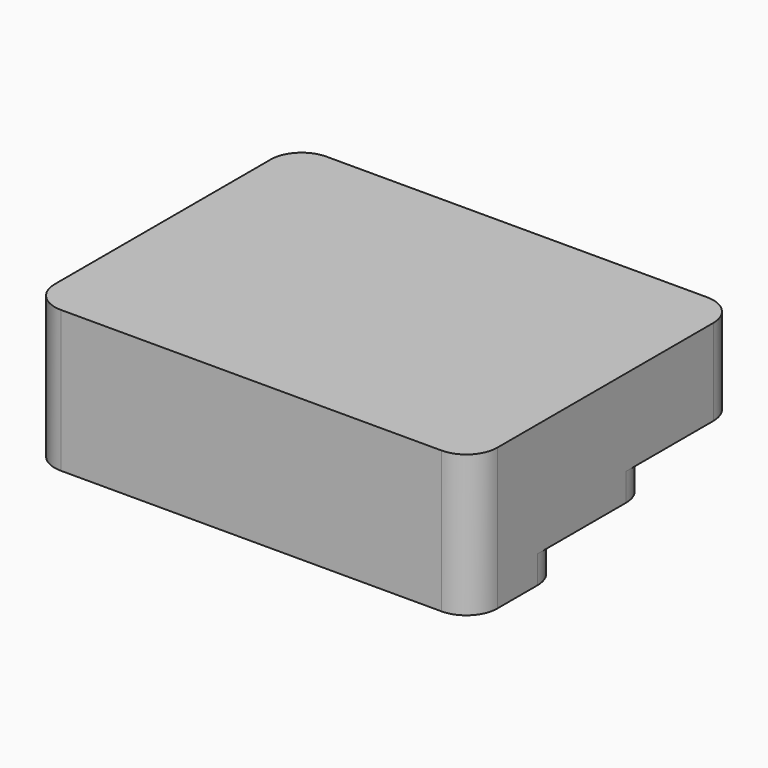
from build123d import *

# Parameters (mm, degrees)
F0_W     = 160
F0_H     = 120
F0_W_2   = 38.2
F0_H_2   = 38.2
F0_W_3   = 38.8
F0_H_3   = 38.8
F1_DEPTH = 50
F2_W     = 160
F2_H     = 120
F3_DEPTH = 1.2
F5_DEPTH = 160.001
F7_DEPTH = 158.8
F8_R     = 10
F9_R     = 11.2
F10_R    = 10
F11_R    = 11.2
F11_R_2  = 11.19999


# Not quite as in the source:
# - a fillet or chamfer is up to 0.001 mm smaller than in the source, because OpenCascade refuses the exact size


with BuildPart() as f1:
    # F0 (on Top) → F1 (new body)
    with BuildSketch(Plane.XY):
        with Locations((-80, -60)):
            Rectangle(F0_W, F0_H)
        with Locations((-139.7, -99.7)):
            Rectangle(F0_W_2, F0_H_2, mode=Mode.SUBTRACT)
        with Locations((-100, -99.7)):
            Rectangle(F0_W_3, F0_H_2, mode=Mode.SUBTRACT)
        with Locations((-60, -99.7)):
            Rectangle(F0_W_3, F0_H_2, mode=Mode.SUBTRACT)
        with Locations((-20.3, -99.7)):
            Rectangle(F0_W_2, F0_H_2, mode=Mode.SUBTRACT)
        with Locations((-139.7, -60)):
            Rectangle(F0_W_2, F0_H_3, mode=Mode.SUBTRACT)
        with Locations((-100, -60)):
            Rectangle(F0_W_3, F0_H_3, mode=Mode.SUBTRACT)
        with Locations((-139.7, -20.3)):
            Rectangle(F0_W_2, F0_H_2, mode=Mode.SUBTRACT)
        with Locations((-100, -20.3)):
            Rectangle(F0_W_3, F0_H_2, mode=Mode.SUBTRACT)
        with Locations((-60, -60)):
            Rectangle(F0_W_3, F0_H_3, mode=Mode.SUBTRACT)
        with Locations((-20.3, -60)):
            Rectangle(F0_W_2, F0_H_3, mode=Mode.SUBTRACT)
        with Locations((-60, -20.3)):
            Rectangle(F0_W_3, F0_H_2, mode=Mode.SUBTRACT)
        with Locations((-20.3, -20.3)):
            Rectangle(F0_W_2, F0_H_2, mode=Mode.SUBTRACT)
    extrude(amount=F1_DEPTH)

    # F2 (on face) → F3 (join)
    with BuildSketch(Plane.XY.offset(50)):
        with Locations((-80, -60)):
            Rectangle(F2_W, F2_H)
    extrude(amount=F3_DEPTH)

    # F4 (on face) → F5 (cut, through all)
    with BuildSketch(Plane(origin=(-160, 0, 0), x_dir=(0, -1, 0), z_dir=(-1, 0, 0))):
        Polygon((79.4, 0), (79.4, 10), (39.4, 10), (39.4, 20), (0, 20), (0, 0), align=None)
    extrude(amount=-F5_DEPTH, mode=Mode.SUBTRACT)

    # F6 (on face) → F7 (join, through all)
    with BuildSketch(Plane(origin=(-160, 0, 0), x_dir=(0, -1, 0), z_dir=(-1, 0, 0))):
        Polygon((40.6, 50), (40.6, 41.2), (79.4, 41.2), (79.4, 31.2), (118.8, 31.2), (118.8, 50), align=None)
    extrude(amount=-F7_DEPTH)

    # F8
    f8_edges = [f1.edges().sort_by_distance(p)[0] for p in [
        (-1.2, -118.8, 15.6),
        (-1.2, -1.2, 35),
        (-158.8, -118.8, 15.6),
        (-158.8, -1.2, 35),
    ]]
    fillet(f8_edges, radius=F8_R)

    # F9
    f9_edges = [f1.edges().sort_by_distance(p)[0] for p in [
        (-160, 0, 35.6),
        (0, 0, 35.6),
        (0, -120, 25.6),
        (-160, -120, 25.6),
    ]]
    fillet(f9_edges, radius=F9_R)

    # F10
    f10_edges = [f1.edges().sort_by_distance(p)[0] for p in [
        (-158.8, -80.6, 15.6),
        (-158.8, -40.6, 25.6),
        (-1.2, -40.6, 25.6),
        (-1.2, -80.6, 15.6),
    ]]
    fillet(f10_edges, radius=F10_R)

    # F11 (call 1 of 4: OpenCascade refuses the feature's edges together)
    f11_edges = [f1.edges().sort_by_distance(p)[0] for p in [
        (-160, -79.4, 5),
    ]]
    fillet(f11_edges, radius=F11_R)

    # F11#2 (call 2 of 4)
    f11_2_edges = [f1.edges().sort_by_distance(p)[0] for p in [
        (-160, -39.4, 15),
    ]]
    fillet(f11_2_edges, radius=F11_R)

    # F11#3 (call 3 of 4) (radius 11.2 in the source; OpenCascade refuses exactly that, so slightly less here)
    f11_3_edges = [f1.edges().sort_by_distance(p)[0] for p in [
        (0, -79.4, 5),
    ]]
    fillet(f11_3_edges, radius=F11_R_2)

    # F11#4 (call 4 of 4)
    f11_4_edges = [f1.edges().sort_by_distance(p)[0] for p in [
        (0, -39.4, 15),
    ]]
    fillet(f11_4_edges, radius=F11_R)


solid = f1.part
